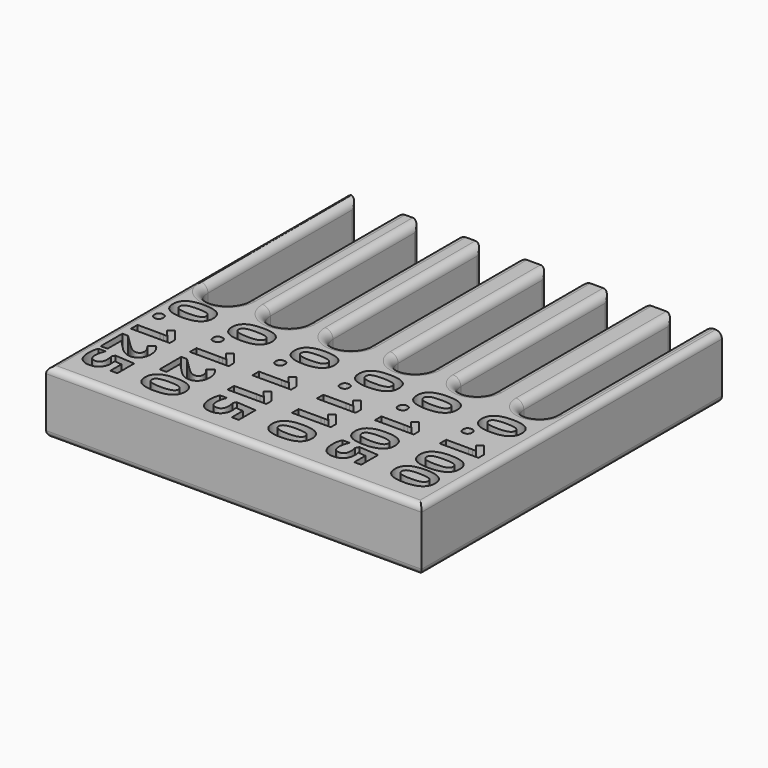
from build123d import *

# Parameters (mm, degrees)
F1_DEPTH     = 5.08
F2_R         = 0.635
F3_T1_DEPTH  = 33.02
F3_T3_DEPTH  = 33.02
F4_TEXT_SIZE = 4.4097222222
F5_DEPTH     = 25.4


# Not quite as in the source:
# - a fillet or chamfer that OpenCascade refuses, or shapes differently, is made with other operations: its cross-section is extruded or revolved along the edge and cut away or added
# - Text() gives the source's letters only with a copy of the font that has no kerning and outlines rounded to 1/6400 em; it was checked with that copy


with BuildPart() as f1:
    # F0 (on Top) → F1 (new body)
    with BuildSketch(Plane.XY):
        with BuildLine():
            Line((2.54, -15.24), (2.54, 15.24))
            Line((2.54, 15.24), (1.5875, 15.24))
            Line((1.5875, 15.24), (1.5875, 0))
            ThreePointArc((1.5875, 0), (0, -1.5875), (-1.5875, 0))
            Line((-1.5875, 0), (-1.5875, 15.24))
            Line((-1.5875, 15.24), (-2.54, 15.24))
            Line((-2.54, 15.24), (-2.54, -15.24))
            Line((-2.54, -15.24), (2.54, -15.24))
        make_face()
        with BuildLine():
            Line((3.4735886571, 15.24), (2.54, 15.24))
            Line((2.54, 15.24), (2.54, -15.24))
            Line((2.54, -15.24), (7.62, -15.24))
            Line((7.62, -15.24), (7.62, 15.24))
            Line((7.62, 15.24), (6.5215886571, 15.24))
            Line((6.5215886571, 15.24), (6.5215886571, 0))
            ThreePointArc((6.5215886571, 0), (4.9975886571, -1.524), (3.4735886571, 0))
            Line((3.4735886571, 0), (3.4735886571, 15.24))
        make_face()
        with BuildLine():
            Line((7.62, 15.24), (7.62, -15.24))
            Line((7.62, -15.24), (12.7, -15.24))
            Line((12.7, -15.24), (12.7, 15.24))
            Line((12.7, 15.24), (11.4789613224, 15.24))
            Line((11.4789613224, 15.24), (11.4789613224, 0))
            ThreePointArc((11.4789613224, 0), (10.0184613224, -1.4605), (8.5579613224, 0))
            Line((8.5579613224, 0), (8.5579613224, 15.24))
            Line((8.5579613224, 15.24), (7.62, 15.24))
        make_face()
        with BuildLine():
            Line((12.7, 15.24), (12.7, -15.24))
            Line((12.7, -15.24), (17.78, -15.24))
            Line((17.78, -15.24), (17.78, 15.24))
            Line((17.78, 15.24), (16.637, 15.24))
            Line((16.637, 15.24), (16.637, 0))
            ThreePointArc((16.637, 0), (15.24, -1.397), (13.843, 0))
            Line((13.843, 0), (13.843, 15.24))
            Line((13.843, 15.24), (12.7, 15.24))
        make_face()
        with BuildLine():
            Line((17.78, 15.24), (17.78, -15.24))
            Line((17.78, -15.24), (22.86, -15.24))
            Line((22.86, -15.24), (22.86, 15.24))
            Line((22.86, 15.24), (21.6034259647, 15.24))
            Line((21.6034259647, 15.24), (21.6034259647, 0))
            ThreePointArc((21.6034259647, 0), (20.2699259647, -1.3335), (18.9364259647, 0))
            Line((18.9364259647, 0), (18.9364259647, 15.24))
            Line((18.9364259647, 15.24), (17.78, 15.24))
        make_face()
        with BuildLine():
            Line((22.86, 15.24), (22.86, -15.24))
            Line((22.86, -15.24), (27.94, -15.24))
            Line((27.94, -15.24), (27.94, 15.24))
            Line((27.94, 15.24), (26.5944115818, 15.24))
            Line((26.5944115818, 15.24), (26.5944115818, 0))
            ThreePointArc((26.5944115818, 0), (25.3244115818, -1.27), (24.0544115818, 0))
            Line((24.0544115818, 0), (24.0544115818, 15.24))
            Line((24.0544115818, 15.24), (22.86, 15.24))
        make_face()
    extrude(amount=F1_DEPTH)

    # F2
    f2_edges = [f1.edges().sort_by_distance(p)[0] for p in [
        (0, -1.5875, 5.08),
        (4.997589, -1.524, 5.08),
        (10.018461, -1.4605, 5.08),
        (15.24, -1.397, 5.08),
        (20.269926, -1.3335, 5.08),
        (25.324412, -1.27, 5.08),
        (25.324412, -1.27, 0),
        (20.269926, -1.3335, 0),
        (15.24, -1.397, 0),
        (10.018461, -1.4605, 0),
        (4.997589, -1.524, 0),
        (0, -1.5875, 0),
        (24.054412, 15.24, 2.54),
        (26.594412, 15.24, 2.54),
        (21.603426, 15.24, 2.54),
        (18.936426, 15.24, 2.54),
        (13.843, 15.24, 2.54),
        (8.557961, 15.24, 2.54),
        (3.473589, 15.24, 2.54),
        (-1.5875, 15.24, 2.54),
        (16.637, 15.24, 2.54),
        (11.478961, 15.24, 2.54),
        (6.521589, 15.24, 2.54),
        (1.5875, 15.24, 2.54),
    ]]
    fillet(f2_edges, radius=F2_R)

    # F3: fillet of radius 0.508 on 6 edges, made by hand

    # F3_s2 → F3_t1 (cut)
    with BuildSketch(Plane.XZ.offset(-16.51)):
        with BuildLine():
            ThreePointArc((27.432, 5.08), (27.7912102448, 4.9312102448), (27.94, 4.572))
            Line((27.94, 4.572), (27.95016, 4.572))
            Line((27.95016, 4.572), (27.95016, 5.09016))
            Line((27.95016, 5.09016), (27.432, 5.09016))
            Line((27.432, 5.09016), (27.432, 5.08))
        make_face()
        with BuildLine():
            ThreePointArc((-2.032, 5.08), (-2.3912102448, 4.9312102448), (-2.54, 4.572))
            Line((-2.54, 4.572), (-2.55016, 4.572))
            Line((-2.55016, 4.572), (-2.55016, 5.09016))
            Line((-2.55016, 5.09016), (-2.032, 5.09016))
            Line((-2.032, 5.09016), (-2.032, 5.08))
        make_face()
        with BuildLine():
            ThreePointArc((27.432, 0), (27.7912102448, 0.1487897552), (27.94, 0.508))
            Line((27.94, 0.508), (27.95016, 0.508))
            Line((27.95016, 0.508), (27.95016, -0.01016))
            Line((27.95016, -0.01016), (27.432, -0.01016))
            Line((27.432, -0.01016), (27.432, 0))
        make_face()
        with BuildLine():
            ThreePointArc((-2.032, 0), (-2.3912102448, 0.1487897552), (-2.54, 0.508))
            Line((-2.54, 0.508), (-2.55016, 0.508))
            Line((-2.55016, 0.508), (-2.55016, -0.01016))
            Line((-2.55016, -0.01016), (-2.032, -0.01016))
            Line((-2.032, -0.01016), (-2.032, 0))
        make_face()
    extrude(amount=F3_T1_DEPTH, mode=Mode.SUBTRACT)

    # F3_s4 → F3_t3 (cut)
    with BuildSketch(Plane.YZ.offset(-3.81)):
        with BuildLine():
            ThreePointArc((-14.732, 5.08), (-15.0912102448, 4.9312102448), (-15.24, 4.572))
            Line((-15.24, 4.572), (-15.25016, 4.572))
            Line((-15.25016, 4.572), (-15.25016, 5.09016))
            Line((-15.25016, 5.09016), (-14.732, 5.09016))
            Line((-14.732, 5.09016), (-14.732, 5.08))
        make_face()
        with BuildLine():
            ThreePointArc((-14.732, 0), (-15.0912102448, 0.1487897552), (-15.24, 0.508))
            Line((-15.24, 0.508), (-15.25016, 0.508))
            Line((-15.25016, 0.508), (-15.25016, -0.01016))
            Line((-15.25016, -0.01016), (-14.732, -0.01016))
            Line((-14.732, -0.01016), (-14.732, 0))
        make_face()
    extrude(amount=F3_T3_DEPTH, mode=Mode.SUBTRACT)

    # F4 (on face) → F5 (cut)
    with BuildSketch(Plane.XY.offset(5.08)):
        with Locations(Location((-1.5875, -2.2225), (0, 0, -90))):
            Text('0.125', F4_TEXT_SIZE, font='Open Sans', font_style=FontStyle.BOLD, text_align=(TextAlign.LEFT, TextAlign.BOTTOM))
        with Locations(Location((3.3162938006, -2.3774872104), (0, 0, -90))):
            Text('0.120', F4_TEXT_SIZE, font='Open Sans', font_style=FontStyle.BOLD, text_align=(TextAlign.LEFT, TextAlign.BOTTOM))
        with Locations(Location((8.4197496571, -2.4148241653), (0, 0, -90))):
            Text('0.115', F4_TEXT_SIZE, font='Open Sans', font_style=FontStyle.BOLD, text_align=(TextAlign.LEFT, TextAlign.BOTTOM))
        with Locations(Location((13.5989485815, -2.3491245317), (0, 0, -90))):
            Text('0.110', F4_TEXT_SIZE, font='Open Sans', font_style=FontStyle.BOLD, text_align=(TextAlign.LEFT, TextAlign.BOTTOM))
        with Locations(Location((18.3287598193, -2.3694505951), (0, 0, -90))):
            Text('0.105', F4_TEXT_SIZE, font='Open Sans', font_style=FontStyle.BOLD, text_align=(TextAlign.LEFT, TextAlign.BOTTOM))
        with Locations(Location((23.5400636256, -2.3067623413), (0, 0, -90))):
            Text('0.100', F4_TEXT_SIZE, font='Open Sans', font_style=FontStyle.BOLD, text_align=(TextAlign.LEFT, TextAlign.BOTTOM))
    extrude(amount=-F5_DEPTH, mode=Mode.SUBTRACT)


solid = f1.part
